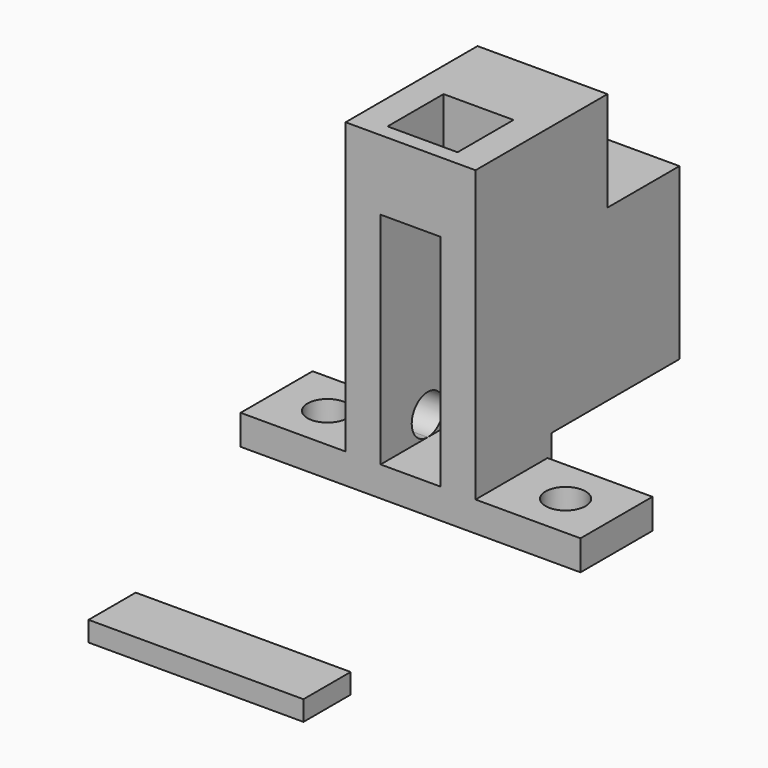
from build123d import *

# Parameters (mm, degrees)
F0_W      = 13
F0_H      = 25.5
F1_DEPTH  = 32
F2_W      = 7
F2_H      = 7
F3_DEPTH  = 7
F4_W      = 6
F4_H      = 2.3767555878
F5_DEPTH  = 25
F2_W_2    = 13
F2_H_2    = 9
F6_DEPTH  = 10
F7_W      = 10.5
F7_H      = 9
F7_R      = 2
F7_W_2    = 13
F8_DEPTH  = 3
F7_H_2    = 16
F9_DEPTH  = 5
F11_DEPTH = 7
F12_W     = 21.5
F12_H     = 5.9
F13_DEPTH = 2


# Not quite as in the source:
# - a feature names something its author has since deleted; it is built from what else it names


with BuildPart() as f1:
    # F0 (on Top) → F1 (new body)
    with BuildSketch(Plane.XY):
        with Locations((0, 7.75)):
            Rectangle(F0_W, F0_H)
    extrude(amount=F1_DEPTH)

    # F2 (on face) → F3 (cut)
    with BuildSketch(Plane.XY.offset(32)):
        Rectangle(F2_W, F2_H)
    extrude(amount=-F3_DEPTH, mode=Mode.SUBTRACT)

    # F4 (on face) → F5 (cut)
    with BuildSketch(Plane.XY):
        Polygon((3, 3), (-3, 3), (-3, -3), (-3, -5), (3, -5), (3, -3), align=None)
        with Locations((0, -6.1883777939)):
            Rectangle(F4_W, F4_H)
    extrude(amount=F5_DEPTH, mode=Mode.SUBTRACT)

    # F2 (on face) → F6 (cut)
    with BuildSketch(Plane.XY.offset(32)):
        with Locations((0, 16)):
            Rectangle(F2_W_2, F2_H_2)
    extrude(amount=-F6_DEPTH, mode=Mode.SUBTRACT)

    # F7 (on face) → F8 (join)
    with BuildSketch(Plane.XY):
        with Locations((11.75, -0.5)):
            Rectangle(F7_W, F7_H)
        with Locations((11.9080794975, -0.5)):
            Circle(F7_R, mode=Mode.SUBTRACT)
        with Locations((-11.75, -0.5)):
            Rectangle(F7_W, F7_H)
        with Locations((-11.9080794975, -0.5)):
            Circle(F7_R, mode=Mode.SUBTRACT)
        with Locations((0, -0.5)):
            Rectangle(F7_W_2, F7_H)
    extrude(amount=F8_DEPTH)

    # F7 (on face) → F9 (cut)
    with BuildSketch(Plane.XY):
        Polygon((-8.2614710554, 4.5), (-6.5, 4.5), (-6.5, 20.5), (6.5, 20.5), (6.5, 4.5), (7.7385289446, 4.5), (7.7385289446, 22.5), (-8.2614710554, 22.5), align=None)
        with Locations((0, 12.5)):
            Rectangle(F7_W_2, F7_H_2)
    extrude(amount=F9_DEPTH, mode=Mode.SUBTRACT)

    # F10 (on face) → F11 (cut)
    with BuildSketch(Plane(origin=(-6.5, 0, 0), x_dir=(0, -1, 0), z_dir=(-1, 0, 0))):
        with BuildLine():
            ThreePointArc((-0.8941277629, 3), (0.5200857995, 3.5857864376), (1.1058722371, 5))
            ThreePointArc((1.1058722371, 5), (-2.3083413252, 6.4142135624), (-0.8941277629, 3))
        make_face()
    extrude(amount=-F11_DEPTH, mode=Mode.SUBTRACT)


with BuildPart() as f13:
    # F12 (on Top) → F13 (new body)
    with BuildSketch(Plane.XY):
        with Locations((5.1557905699, -35.3235676074)):
            Rectangle(F12_W, F12_H)
    extrude(amount=F13_DEPTH)


solid = Compound([f1.part, f13.part])
